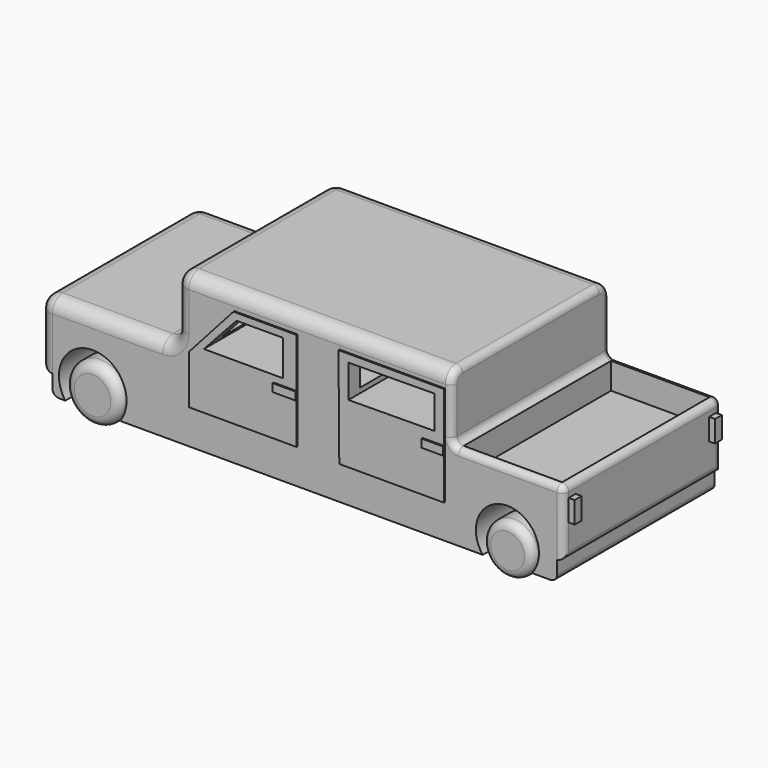
from build123d import *

# Parameters (mm, degrees)
F0_W          = 202.681414783
F0_H          = 76.2539217249
F1_DEPTH      = 25.4
F2_W          = 106.77928105
F2_H          = 76.2539217249
F3_DEPTH      = 25.4
F4_F1_R       = 5.08
F4_F2_R       = 5.08
F5_F1_R       = 2.54
F5_F2_R       = 2.54
F6_R          = 2.54
F7_W          = 195.061414783
F7_H          = 76.2539217249
F8_DEPTH      = 7.62
F9_R          = 2.54
F11_T1_DEPTH  = 101.69928105
F11_S5_W      = 5.08
F11_S5_H      = 5.08
F11_T6_DEPTH  = 5.08
F11_T10_ANGLE = 90
F11_T12_ANGLE = 90
F11_S15_W     = 5.08
F11_S15_H     = 5.08
F11_T16_DEPTH = 5.08
F13_R         = 11.0657503551
F13_R_2       = 11.0164771161
F16_DEPTH     = 78.74
F15_W         = 38.0459423494
F15_H         = 71.1739217249
F17_DEPTH     = 10.16
F18_W         = 6.7701749504
F18_H         = 2.1561356261
F19_DEPTH     = 0.508
F20_W         = 9.2535796575
F20_H         = 2.0127247553
F20_W_2       = 5.8551989496
F20_H_2       = 1.9212367479
F21_DEPTH     = 0.508
F22_W         = 7.3190014809
F22_H         = 2.1957003046
F23_DEPTH     = 0.508
F24_W         = 6.7700743675
F24_H         = 2.1042132284
F25_DEPTH     = 0.508
F27_DEPTH     = 0.508
F28_W         = 8.7955649942
F28_H         = 3.0446203891
F29_DEPTH     = 0.508
F30_W         = 8.3197318017
F30_H         = 3.1305747107
F31_DEPTH     = 0.508
F33_DEPTH     = 101.346
F34_W         = 3.3496206319
F34_H         = 8.3715431392
F34_W_2       = 3.3222434735
F35_DEPTH     = 2.286
F36_W         = 11.1564658582
F36_H         = 2.4489806965
F36_W_2       = 10.6122493744
F37_DEPTH     = 1.27
F38_DEPTH     = 0.508
F40_DEPTH     = 85.852
F42_DEPTH     = 88.138
F43_R         = 13.0611638595
F43_R_2       = 12.2018746914
F44_DEPTH     = 84.328
F45_R         = 10.7155693868
F46_DEPTH     = 11.938
F45_R_2       = 9.5947246811
F47_R         = 3.6792614691
F48_R         = 3.0660512242
F49_R         = 3.3084211886
F50_DEPTH     = 55.372
F51_R         = 10.1042496204
F52_DEPTH     = 10.16
F51_R_2       = 10.9006597161
F53_R         = 3.0734
F54_R         = 3.0734
F55_R         = 3.8095425569
F56_DEPTH     = 54.864


# Not quite as in the source:
# - a fillet or chamfer that OpenCascade refuses, or shapes differently, is made with other operations: its cross-section is extruded or revolved along the edge and cut away or added


with BuildPart() as f1:
    # F0 (on Top) → F1 (new body)
    with BuildSketch(Plane.XY):
        with Locations((-2.5283508003, 22.6992699318)):
            Rectangle(F0_W, F0_H)
    extrude(amount=F1_DEPTH)

    # F2 (on face) → F3 (join)
    with BuildSketch(Plane.XY.offset(25.4)):
        with Locations((2.2967737168, 22.6992699318)):
            Rectangle(F2_W, F2_H)
    extrude(amount=F3_DEPTH)

    # F4: fillet of radius 5.08 on 8 edges, made by hand

    # F4_f1
    f4_f1_edges = [f1.edges().sort_by_distance(p)[0] for p in [
        (-51.0928668082, 22.6992699318, 25.4),
    ]]
    fillet(f4_f1_edges, radius=F4_F1_R)

    # F4_f2
    f4_f2_edges = [f1.edges().sort_by_distance(p)[0] for p in [
        (-51.0928668082, 22.6992699318, 50.8),
        (-51.0928668082, 60.8262307942, 40.64),
        (-51.0928668082, -15.4276909307, 40.64),
        (-103.8690581918, 22.6992699318, 25.4),
        (-103.8690581918, 60.8262307942, 12.7),
        (-103.8690581918, -15.4276909307, 12.7),
        (-103.8690581918, 22.6992699318, 0),
        (-52.5807643597, -15.4276909307, 26.8878975516),
        (-52.5807643597, 60.8262307942, 26.8878975516),
    ]]
    fillet(f4_f2_edges, radius=F4_F2_R)

    # F5: fillet of radius 2.54 on 4 edges, made by hand

    # F5_f1
    f5_f1_edges = [f1.edges().sort_by_distance(p)[0] for p in [
        (55.6864142418, 22.6992699318, 25.4),
    ]]
    fillet(f5_f1_edges, radius=F5_F1_R)

    # F5_f2
    f5_f2_edges = [f1.edges().sort_by_distance(p)[0] for p in [
        (55.6864142418, 22.6992699318, 50.8),
        (55.6864142418, -15.4276909307, 39.37),
        (55.6864142418, 60.8262307942, 39.37),
        (56.4303630176, 60.8262307942, 26.1439487758),
        (56.4303630176, -15.4276909307, 26.1439487758),
    ]]
    fillet(f5_f2_edges, radius=F5_F2_R)

    # F6
    f6_edges = [f1.edges().sort_by_distance(p)[0] for p in [
        (98.812357, 60.826231, 11.43),
        (98.812357, -15.427691, 11.43),
        (98.812357, -14.683742, 24.656051),
        (98.812357, 22.69927, 0),
        (98.812357, 22.69927, 25.4),
        (98.812357, 60.082282, 24.656051),
    ]]
    fillet(f6_edges, radius=F6_R)

    # F7 (on face) → F8 (join)
    with BuildSketch(Plane(origin=(0, 0, 0), x_dir=(1, 0, 0), z_dir=(0, 0, -1))):
        with Locations((-1.2583508003, -22.6992699318)):
            Rectangle(F7_W, F7_H)
    extrude(amount=F8_DEPTH)

    # F9
    f9_edges = [f1.edges().sort_by_distance(p)[0] for p in [
        (-98.789058, 22.69927, -7.62),
        (-103.869058, 22.69927, 5.08),
        (96.272357, 22.69927, -7.62),
    ]]
    fillet(f9_edges, radius=F9_R)

    # F11: fillet of radius 5.08 on 2 edges, made by hand

    # F11_s2 → F11_t1 (cut)
    with BuildSketch(Plane.YZ.offset(-46.0128668082)):
        with BuildLine():
            ThreePointArc((60.8262307942, 45.72), (59.3383332426, 49.3121024484), (55.7462307942, 50.8))
            Line((55.7462307942, 50.8), (60.8262307942, 50.8))
            Line((60.8262307942, 50.8), (60.8262307942, 45.72))
        make_face()
        with BuildLine():
            ThreePointArc((-10.3476909307, 50.8), (-13.9397933791, 49.3121024484), (-15.4276909307, 45.72))
            Line((-15.4276909307, 45.72), (-15.4276909307, 50.8))
            Line((-15.4276909307, 50.8), (-10.3476909307, 50.8))
        make_face()
    extrude(amount=F11_T1_DEPTH, mode=Mode.SUBTRACT)


with BuildPart() as f11_tool4:
    # F11_s5 → F11_t6 (new body)
    with BuildSketch(Plane.XY.offset(45.72)):
        with Locations((-48.5528668082, -12.8876909307)):
            Rectangle(F11_S5_W, F11_S5_H)
    extrude(amount=F11_T6_DEPTH)

    # F11_s7 → F11_t8 (revolve, cut)
    with BuildSketch(Plane(origin=(-46.0128668082, -10.3476909307, 45.72), x_dir=(0.7071067812, 0.7071067812, 0), z_dir=(0.7071067812, -0.7071067812, 0))):
        with BuildLine():
            ThreePointArc((0, -5.08), (5.08, 0), (0, 5.08))
            Line((0, 5.08), (0, -5.08))
        make_face()
    revolve(axis=Axis((-46.0128668082, -10.3476909307, 45.72), (0, 0, 1)), mode=Mode.SUBTRACT)


with BuildPart() as f1_1:
    add(f1.part)

    # F11_t3: cut F11_tool4
    add(f11_tool4.part, mode=Mode.SUBTRACT)

    # F11_s9 → F11_t10 (revolve, cut)
    with BuildSketch(Plane.XZ.offset(10.3476909307)):
        with BuildLine():
            ThreePointArc((55.6864142418, 48.26), (54.942465466, 50.0560512242), (53.1464142418, 50.8))
            Line((53.1464142418, 50.8), (55.6864142418, 50.8))
            Line((55.6864142418, 50.8), (55.6864142418, 48.26))
        make_face()
    revolve(axis=Axis((55.6864142418, -10.3476909307, 45.72), (1, 0, 0)), revolution_arc=F11_T10_ANGLE, mode=Mode.SUBTRACT)

    # F11_s11 → F11_t12 (revolve, cut)
    with BuildSketch(Plane.XY.offset(45.72)):
        with BuildLine():
            ThreePointArc((55.6864142418, 58.2862307942), (54.942465466, 60.0822820184), (53.1464142418, 60.8262307942))
            Line((53.1464142418, 60.8262307942), (55.6864142418, 60.8262307942))
            Line((55.6864142418, 60.8262307942), (55.6864142418, 58.2862307942))
        make_face()
    revolve(axis=Axis((55.6864142418, 55.7462307942, 45.72), (1, 0, 0)), revolution_arc=F11_T12_ANGLE, mode=Mode.SUBTRACT)


with BuildPart() as f11_tool14:
    # F11_s15 → F11_t16 (new body)
    with BuildSketch(Plane.XZ.offset(-55.7462307942)):
        with Locations((-48.5528668082, 48.26)):
            Rectangle(F11_S15_W, F11_S15_H)
    extrude(amount=-F11_T16_DEPTH)

    # F11_s17 → F11_t18 (revolve, cut)
    with BuildSketch(Plane(origin=(-46.0128668082, 55.7462307942, 45.72), x_dir=(0.7071067812, 0, -0.7071067812), z_dir=(0.7071067812, 0, 0.7071067812))):
        with BuildLine():
            ThreePointArc((0, -5.08), (5.08, 0), (0, 5.08))
            Line((0, 5.08), (0, -5.08))
        make_face()
    revolve(axis=Axis((-46.0128668082, 55.7462307942, 45.72), (0, 1, 0)), mode=Mode.SUBTRACT)


with BuildPart() as f1_2:
    add(f1_1.part)

    # F11_t13: cut F11_tool14
    add(f11_tool14.part, mode=Mode.SUBTRACT)

    # F13 (on face) → F16 (cut)
    with BuildSketch(Plane.XZ.offset(15.4276909307)):
        with Locations((-83.6574137211, 0)):
            Circle(F13_R)
        with Locations((76.5930116177, 0)):
            Circle(F13_R_2)
    extrude(amount=-F16_DEPTH, mode=Mode.SUBTRACT)

    # F15 (on face) → F17 (cut)
    with BuildSketch(Plane.XY.offset(25.4)):
        with Locations((77.2493854165, 22.6992699318)):
            Rectangle(F15_W, F15_H)
    extrude(amount=-F17_DEPTH, mode=Mode.SUBTRACT)

    # F18 (on face) → F19 (join)
    with BuildSketch(Plane.XZ.offset(15.4276909307)):
        Polygon((12.2288102284, 44.2769639194), (12.5434109941, 5.6152399629), (53.0108846724, 5.6152399629), (53.0108846724, 22.789966315), (46.240709722, 22.789966315), (46.240709722, 24.9461019412), (53.0108846724, 24.9461019412), (53.0108846724, 44.2769639194), align=None)
        with Locations((49.6257971972, 23.8680341281)):
            Rectangle(F18_W, F18_H)
    extrude(amount=F19_DEPTH)

    # F20 (on face) → F21 (join)
    with BuildSketch(Plane(origin=(0, 60.8262307942, 0), x_dir=(-1, 0, 0), z_dir=(0, 1, 0))):
        Polygon((47.1537970006, 4.2073712684), (47.1537970006, 25.066524744), (28.8562942296, 44.0959297121), (6.4285122789, 44.0959297121), (6.4285122789, 26.1643752456), (15.6820919365, 26.1643752456), (15.6820919365, 24.1516504902), (6.4285122789, 24.1516504902), (6.4285122789, 4.2073712684), align=None)
        with Locations((11.0553021077, 25.1580128679)):
            Rectangle(F20_W, F20_H)
        Polygon((-14.5087884739, 4.3903472833), (-14.5087884739, 44.0959297121), (-52.3846186697, 44.0959297121), (-52.3846186697, 26.1643752456), (-46.5294197202, 26.1643752456), (-46.5294197202, 24.2431384977), (-52.3846186697, 24.2431384977), (-52.3846186697, 4.3903472833), align=None)
        with Locations((-49.457019195, 25.2037568716)):
            Rectangle(F20_W_2, F20_H_2)
    extrude(amount=F21_DEPTH)

    # F22 (on face) → F23 (join)
    with BuildSketch(Plane(origin=(0, 61.3342307942, 0), x_dir=(-1, 0, 0), z_dir=(0, 1, 0))):
        with Locations((10.0880130194, 23.0538003379)):
            Rectangle(F22_W, F22_H)
    extrude(amount=F23_DEPTH)

    # F24 (on face) → F25 (join)
    with BuildSketch(Plane(origin=(0, 61.3342307942, 0), x_dir=(-1, 0, 0), z_dir=(0, 1, 0))):
        with Locations((-48.999581486, 23.1910318835)):
            Rectangle(F24_W, F24_H)
    extrude(amount=F25_DEPTH)

    # F26 (on face) → F27 (join)
    with BuildSketch(Plane.XZ.offset(15.4276909307)):
        Polygon((-28.3797085285, 44.1427379847), (-45.5197878182, 24.9729100615), (-45.5197878182, 6.0286116786), (-4.0227547288, 6.0286116786), (-4.0227547288, 44.1427379847), align=None)
    extrude(amount=F27_DEPTH)

    # F28 (on face) → F29 (join)
    with BuildSketch(Plane.XZ.offset(15.9356909307)):
        with Locations((-8.4205372259, 23.5633646371)):
            Rectangle(F28_W, F28_H)
    extrude(amount=F29_DEPTH)

    # F30 (on face) → F31 (join)
    with BuildSketch(Plane.XZ.offset(15.9356909307)):
        with Locations((48.8510187715, 23.3808145858)):
            Rectangle(F30_W, F30_H)
    extrude(amount=F31_DEPTH)

    # F33 (cut): a face of the model
    f33_faces = [f1_2.faces().sort_by_distance(p)[0] for p in [
        (-51.0928668082, 22.6992699318, 38.1),
    ]]
    extrude(f33_faces, amount=-F33_DEPTH, mode=Mode.SUBTRACT)

    # F34 (on face) → F35 (join)
    with BuildSketch(Plane.YZ.offset(98.8123565912)):
        with Locations((-11.2128806147, 16.7180355638)):
            Rectangle(F34_W, F34_H)
        with Locations((56.6251090574, 16.7180355638)):
            Rectangle(F34_W_2, F34_H)
    extrude(amount=F35_DEPTH)

    # F36 (on face) → F37 (join)
    with BuildSketch(Plane(origin=(-103.8690581918, 0, 0), x_dir=(0, -1, 0), z_dir=(-1, 0, 0))):
        with Locations((-43.2208161801, 15.0063647889)):
            Rectangle(F36_W, F36_H)
        with Locations((0.0445088372, 15.0063647889)):
            Rectangle(F36_W_2, F36_H)
    extrude(amount=F37_DEPTH)

    # F20 (on face) → F38 (join)
    with BuildSketch(Plane(origin=(0, 60.8262307942, 0), x_dir=(-1, 0, 0), z_dir=(0, 1, 0))):
        Polygon((47.1537970006, 4.2073712684), (47.1537970006, 25.066524744), (28.8562942296, 44.0959297121), (6.4285122789, 44.0959297121), (6.4285122789, 26.1643752456), (15.6820919365, 26.1643752456), (15.6820919365, 24.1516504902), (6.4285122789, 24.1516504902), (6.4285122789, 4.2073712684), align=None)
        with Locations((11.0553021077, 25.1580128679)):
            Rectangle(F20_W, F20_H)
        Polygon((-14.5087884739, 4.3903472833), (-14.5087884739, 44.0959297121), (-52.3846186697, 44.0959297121), (-52.3846186697, 26.1643752456), (-46.5294197202, 26.1643752456), (-46.5294197202, 24.2431384977), (-52.3846186697, 24.2431384977), (-52.3846186697, 4.3903472833), align=None)
        with Locations((-49.457019195, 25.2037568716)):
            Rectangle(F20_W_2, F20_H_2)
    extrude(amount=F38_DEPTH)

    # F39 (on face) → F40 (cut)
    with BuildSketch(Plane.XZ.offset(15.9356909307)):
        Polygon((-27.1853841841, 41.4620190859), (-39.8143306375, 27.7187526226), (-9.1705638915, 27.7187526226), (-9.1705638915, 41.4620190859), align=None)
    extrude(amount=-F40_DEPTH, mode=Mode.SUBTRACT)

    # F41 (on face) → F42 (cut)
    with BuildSketch(Plane.XZ.offset(15.9356909307)):
        Polygon((49.3214164409, 41.5467331021), (16.0873290151, 41.2762984633), (16.0873290151, 28.5625585996), (49.4248646853, 28.8338350244), align=None)
    extrude(amount=-F42_DEPTH, mode=Mode.SUBTRACT)

    # F43 (on face) → F44 (cut)
    with BuildSketch(Plane.XZ.offset(15.4276909307)):
        with Locations((-83.191126585, 0)):
            Circle(F43_R)
        with Locations((77.1336778998, 0)):
            Circle(F43_R_2)
    extrude(amount=-F44_DEPTH, mode=Mode.SUBTRACT)


with BuildPart() as f46:
    # F45 (on face) → F46 (new body)
    with BuildSketch(Plane.XZ.offset(15.4276909307)):
        with Locations((-83.2727625966, -2.3678555153)):
            Circle(F45_R)
    extrude(amount=-F46_DEPTH)

    # F47
    f47_edges = [f46.edges().sort_by_distance(p)[0] for p in [
        (-93.988332, -3.489691, -2.367856),
        (-93.988332, -15.427691, -2.367856),
    ]]
    fillet(f47_edges, radius=F47_R)


with BuildPart() as f46b:
    # F45 (on face) → F46, piece 2 (new body)
    with BuildSketch(Plane.XZ.offset(15.4276909307)):
        with Locations((77.1891474724, -3.1107338145)):
            Circle(F45_R_2)
    extrude(amount=-F46_DEPTH)

    # F48
    f48_edges = [f46b.edges().sort_by_distance(p)[0] for p in [
        (67.594423, -3.489691, -3.110734),
        (67.594423, -15.427691, -3.110734),
    ]]
    fillet(f48_edges, radius=F48_R)

    # F49 (on face) → F50 (join)
    with BuildSketch(Plane(origin=(0, -3.4896909307, 0), x_dir=(-1, 0, 0), z_dir=(0, 1, 0))):
        with Locations((-77.1891474724, -3.1107338145)):
            Circle(F49_R)
    extrude(amount=F50_DEPTH)


with BuildPart() as f52:
    # F51 (on face) → F52 (new body)
    with BuildSketch(Plane(origin=(0, 60.8262307942, 0), x_dir=(-1, 0, 0), z_dir=(0, 1, 0))):
        with Locations((-77.0034268498, -2.8709305916)):
            Circle(F51_R)
    extrude(amount=-F52_DEPTH)

    # F53
    f53_edges = [f52.edges().sort_by_distance(p)[0] for p in [
        (87.107676, 60.826231, -2.870931),
        (87.107676, 50.666231, -2.870931),
    ]]
    fillet(f53_edges, radius=F53_R)


with BuildPart() as f52b:
    # F51 (on face) → F52, piece 2 (new body)
    with BuildSketch(Plane(origin=(0, 60.8262307942, 0), x_dir=(-1, 0, 0), z_dir=(0, 1, 0))):
        with Locations((83.2727625966, -2.3137698881)):
            Circle(F51_R_2)
    extrude(amount=-F52_DEPTH)

    # F54
    f54_edges = [f52b.edges().sort_by_distance(p)[0] for p in [
        (-72.372103, 60.826231, -2.31377),
        (-72.372103, 50.666231, -2.31377),
    ]]
    fillet(f54_edges, radius=F54_R)


with BuildPart() as f56:
    # F55 (on face) → F56 (new body)
    with BuildSketch(Plane(origin=(0, -3.4896909307, 0), x_dir=(-1, 0, 0), z_dir=(0, 1, 0))):
        with Locations((83.2727625966, -2.3678555153)):
            Circle(F55_R)
    extrude(amount=F56_DEPTH)


solid = Compound([f1_2.part, f46.part, f46b.part, f52.part, f52b.part, f56.part])
